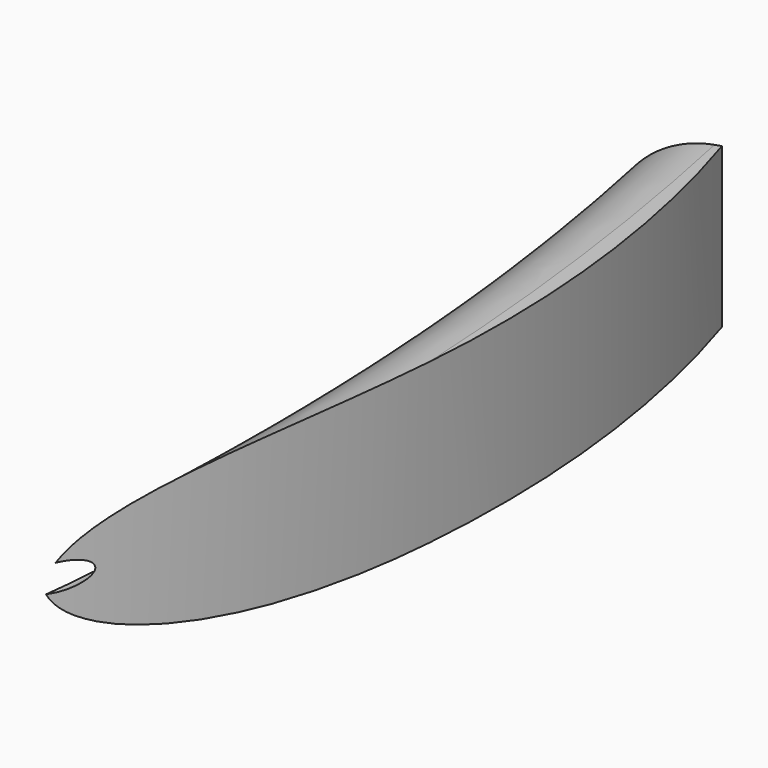
from build123d import *

# Parameters (mm, degrees)
F1_DEPTH    = 7
F2_T2_ANGLE = 26.471202853
F2_T4_ANGLE = 26.471202853
F3_R        = 0.5765318272
F4_DEPTH    = 81.70182


# Not quite as in the source:
# - a fillet or chamfer that OpenCascade refuses, or shapes differently, is made with other operations: its cross-section is extruded or revolved along the edge and cut away or added


with BuildPart() as f1:
    # F0 (on Top) → F1 (new body)
    with BuildSketch(Plane.XY):
        with BuildLine():
            Line((-55.7133033872, 61.0515810549), (-59.585891664, 59.7469322383))
            ThreePointArc((-59.585891664, 59.7469322383), (-57.3715400132, 43.0123532737), (-57.6495975256, 26.1341966689))
            ThreePointArc((-57.6495975256, 26.1341966689), (-53.4588056212, 43.414181653), (-55.7133033872, 61.0515810549))
        make_face()
    extrude(amount=F1_DEPTH)

    # F2: fillet of radius 3.7881425007 on 2 edges, made by hand

    # F2_s1 → F2_t2 (revolve, cut)
    with BuildSketch(Plane(origin=(-23.8154539079, 80.2322879023, 0), x_dir=(0, 0, 1), z_dir=(-0.2845597835, 0.9586582966, 0))):
        with BuildLine():
            ThreePointArc((3.2118574993, -39.7282571763), (5.8904787496, -38.6187359259), (7, -35.9401146756))
            Line((7, -35.9401146756), (7, -39.7282571763))
            Line((7, -39.7282571763), (3.2118574993, -39.7282571763))
        make_face()
    revolve(axis=Axis((-171.3203362847, 36.4482226677, 7), (0, 0, -1)), revolution_arc=F2_T2_ANGLE, mode=Mode.SUBTRACT)

    # F2_s3 → F2_t4 (revolve, cut)
    with BuildSketch(Plane(origin=(-23.8154539079, 80.2322879023, 0), x_dir=(0, 0, 1), z_dir=(-0.2845597835, 0.9586582966, 0))):
        with BuildLine():
            ThreePointArc((3.7881425007, -39.7282571763), (1.1095212504, -38.6187359259), (0, -35.9401146756))
            Line((0, -35.9401146756), (0, -39.7282571763))
            Line((0, -39.7282571763), (3.7881425007, -39.7282571763))
        make_face()
    revolve(axis=Axis((-171.3203362847, 36.4482226677, 0), (0, 0, -1)), revolution_arc=F2_T4_ANGLE, mode=Mode.SUBTRACT)

    # F3 (on Front) → F4 (cut)
    with BuildSketch(Plane.XZ):
        with Locations((-57.4206672609, 3.7390380166)):
            Circle(F3_R)
    extrude(amount=-F4_DEPTH, mode=Mode.SUBTRACT)


solid = f1.part
